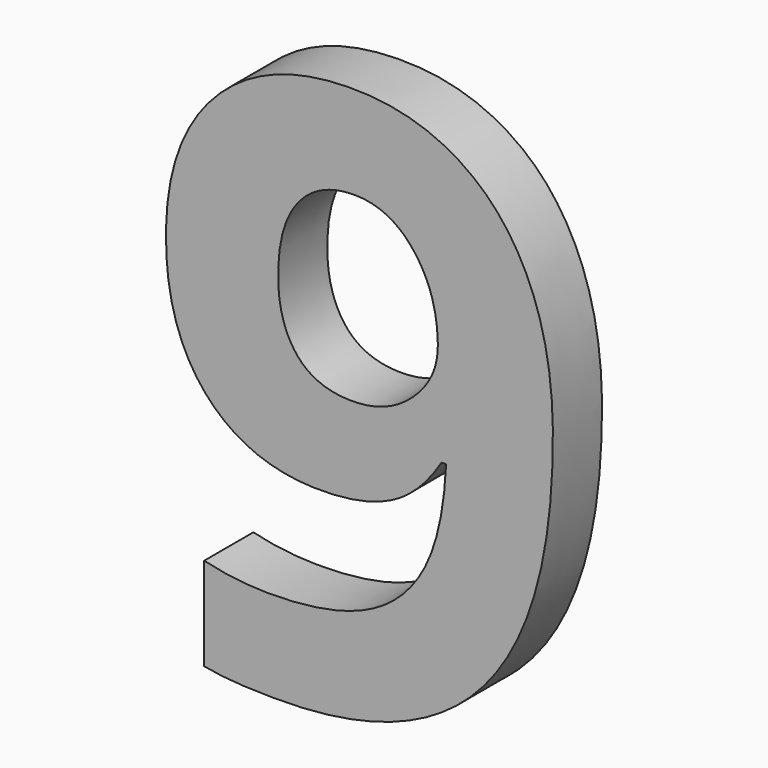
from build123d import *

# Parameters (mm, degrees)
F0_TEXT_SIZE = 62.5
F1_DEPTH     = 5


# Not quite as in the source:
# - Text() gives the source's letters only with a copy of the font that has no kerning and outlines rounded to 1/6400 em; it was checked with that copy


with BuildPart() as f1:
    # F0 (on Front) → F1 (new body)
    with BuildSketch(Plane.XZ):
        with Locations((-57.3898729945, 12.9845819773)):
            Text('9', F0_TEXT_SIZE, font='Open Sans', font_style=FontStyle.BOLD, text_align=(TextAlign.LEFT, TextAlign.BOTTOM))
    extrude(amount=F1_DEPTH)


solid = f1.part
